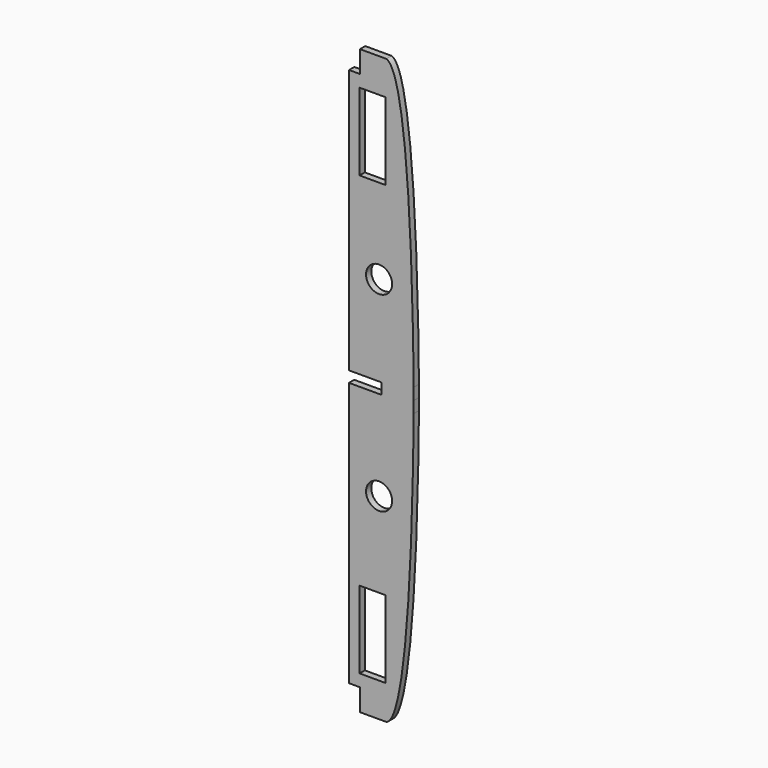
from build123d import *

# Parameters (mm, degrees)
F0_W     = 23.5877633095
F0_H     = 70.452131331
F0_R     = 11.8720680475
F1_DEPTH = 6


# Not quite as in the source:
# - a feature names something its author has since deleted; it is built from what else it names


with BuildPart() as f1:
    # F0 (on Front) → F1 (new body)
    with BuildSketch(Plane.XZ):
        with BuildLine():
            add(Edge.make_bspline(
                [(611.5972634537, -153.9022508941), (611.6433594367, -147.41064865), (611.6495089066, -143.6068529658), (611.6564787513, -143.3067750725)],
                knots=[235.725136676, 235.725136676, 235.725136676, 235.725136676, 267.1722290958, 267.1722290958, 267.1722290958, 267.1722290958], degree=3))
            Line((611.6564787513, -143.3067750725), (582.1564787513, -143.3067750725))
            Line((582.1564787513, -143.3067750725), (582.1564787513, -148.3067750725))
            Line((582.1564787513, -148.3067750725), (552.6564787513, -148.3067750725))
            Line((552.6564787513, -148.3067750725), (552.6564787513, -389.3067750725))
            Line((552.6564787513, -389.3067750725), (562.6564787513, -389.3067750725))
            Line((562.6564787513, -389.3067750725), (562.6564787513, -409.3067750725))
            Line((562.6564787513, -409.3067750725), (586.6564787513, -409.3067750725))
            add(Edge.make_bspline(
                [(586.6564787513, -409.3067750725), (608.6616471129, -402.2484026518), (611.2517312901, -202.5628331126), (611.5972634537, -153.9022508941)],
                knots=[0, 0, 0, 0, 235.725136676, 235.725136676, 235.725136676, 235.725136676], degree=3))
        make_face()
        with Locations((574.0745894078, -343.064654055)):
            Rectangle(F0_W, F0_H, mode=Mode.SUBTRACT)
        with Locations((580.0634622574, -230.3008177464)):
            Circle(F0_R, mode=Mode.SUBTRACT)
        with BuildLine():
            add(Edge.make_bspline(
                [(586.6564787513, 122.6932249275), (608.6616471129, 115.6348525069), (611.2517312901, -84.0507170322), (611.5972634537, -132.7112992508)],
                knots=[0, 0, 0, 0, 235.725136676, 235.725136676, 235.725136676, 235.725136676], degree=3))
            Line((586.6564787513, 122.6932249275), (562.6564787513, 122.6932249275))
            Line((562.6564787513, 122.6932249275), (562.6564787513, 102.6932249275))
            Line((562.6564787513, 102.6932249275), (552.6564787513, 102.6932249275))
            Line((552.6564787513, 102.6932249275), (552.6564787513, -138.3067750725))
            Line((552.6564787513, -138.3067750725), (582.1564787513, -138.3067750725))
            Line((582.1564787513, -138.3067750725), (582.1564787513, -143.3067750725))
            Line((582.1564787513, -143.3067750725), (611.6564787513, -143.3067750725))
            add(Edge.make_bspline(
                [(611.5972634537, -132.7112992508), (611.6433594367, -139.2029014949), (611.6495089066, -143.0066971792), (611.6564787513, -143.3067750725)],
                knots=[235.725136676, 235.725136676, 235.725136676, 235.725136676, 267.1722290958, 267.1722290958, 267.1722290958, 267.1722290958], degree=3))
        make_face()
        with Locations((580.0634622574, -56.3127323985)):
            Circle(F0_R, mode=Mode.SUBTRACT)
        with Locations((574.0745894078, 56.4511039101)):
            Rectangle(F0_W, F0_H, mode=Mode.SUBTRACT)
    extrude(amount=F1_DEPTH)


solid = f1.part
